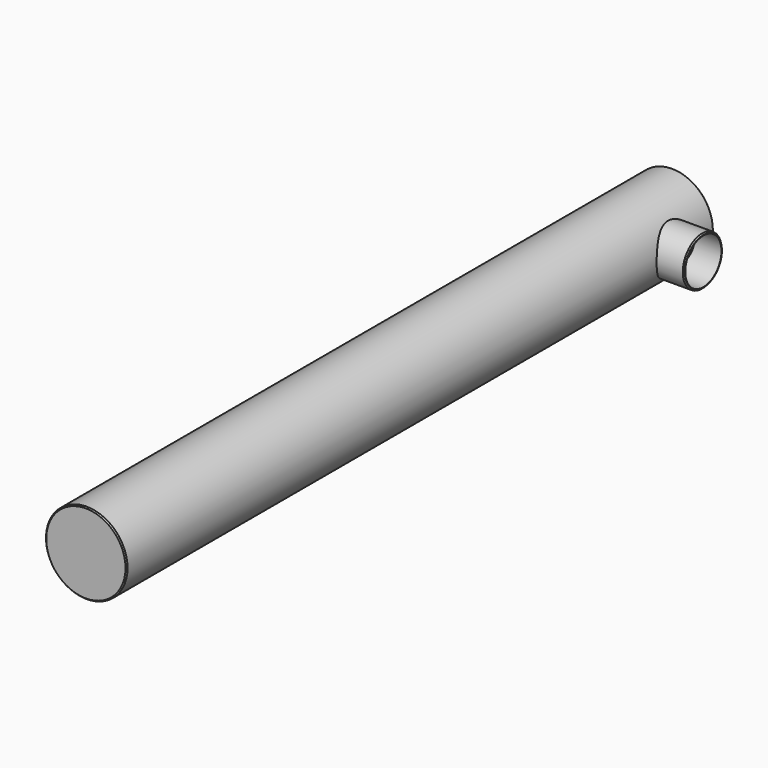
from build123d import *

# Parameters (mm, degrees)
F0_R     = 228.6
F0_R_2   = 222.25
F1_DEPTH = 4114.8
F2_SIZE  = 6.34999
F3_R     = 136.525
F3_R_2   = 127
F4_DEPTH = 25.4
F5_DEPTH = 381
F6_SIZE  = 6.35
F7_SIZE  = 6.34999


# Not quite as in the source:
# - a fillet or chamfer is up to 0.001 mm smaller than in the source, because OpenCascade refuses the exact size


with BuildPart() as f1:
    # F0 (on Front) → F1 (new body)
    with BuildSketch(Plane.XZ):
        Circle(F0_R)
        Circle(F0_R_2, mode=Mode.SUBTRACT)
    extrude(amount=F1_DEPTH)

    # F2 (size 6.35 in the source; OpenCascade refuses exactly that, so slightly less here)
    f2_edges = [f1.edges().sort_by_distance(p)[0] for p in [
        (-228.6, -4114.8, 0),
    ]]
    chamfer(f2_edges, length=F2_SIZE)

    # F7 (size 6.35 in the source; OpenCascade refuses exactly that, so slightly less here)
    f7_edges = [f1.edges().sort_by_distance(p)[0] for p in [
        (-228.6, 0, 0),
    ]]
    chamfer(f7_edges, length=F7_SIZE)


with BuildPart() as f4:
    # F3 (on Right) → F4 (new body)
    with BuildSketch(Plane.YZ):
        with Locations((-263.525, 0)):
            Circle(F3_R)
        with Locations((-263.525, 0)):
            Circle(F3_R_2, mode=Mode.SUBTRACT)
    extrude(amount=F4_DEPTH)


with BuildPart() as f5:
    # F3 (on Right) → F5 (new body)
    with BuildSketch(Plane.YZ):
        with Locations((-263.525, 0)):
            Circle(F3_R)
        with Locations((-263.525, 0)):
            Circle(F3_R_2, mode=Mode.SUBTRACT)
    extrude(amount=F5_DEPTH)

    # F6
    f6_edges = [f5.edges().sort_by_distance(p)[0] for p in [
        (381, -400.05, 0),
    ]]
    chamfer(f6_edges, length=F6_SIZE)


solid = Compound([f1.part, f4.part, f5.part])
